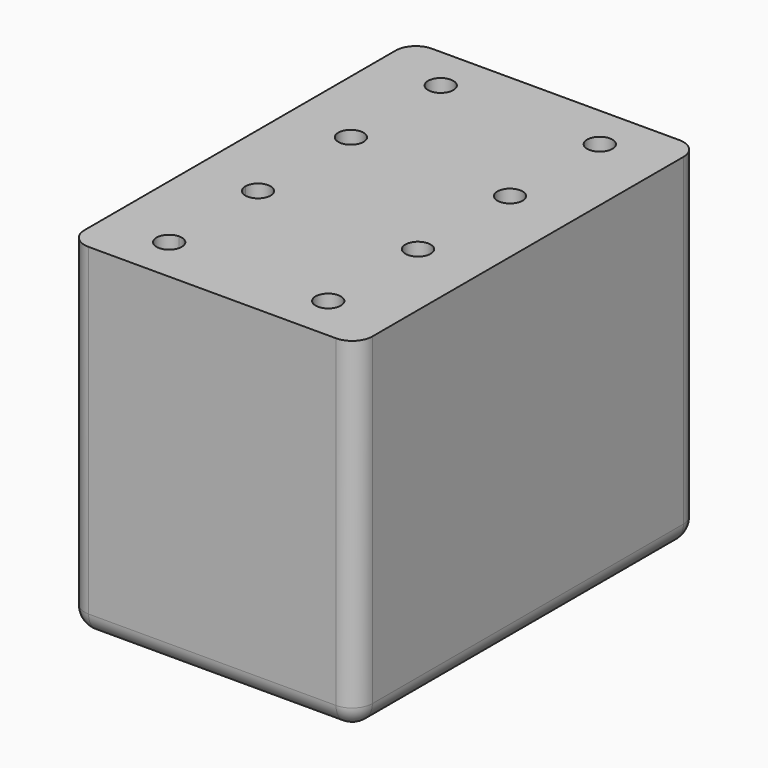
from build123d import *

# Parameters (mm, degrees)
F0_R     = 2.5
F1_DEPTH = 68
F2_R     = 4


with BuildPart() as f1:
    # F0 (on Top) → F1 (new body)
    with BuildSketch(Plane.XY):
        with BuildLine():
            Line((-44.25, -10.5), (-44.25, 0))
            Line((-44.25, 0), (-57, 0))
            Line((-57, 0), (-57, -22))
            Line((-57, -22), (0, -22))
            Line((0, -22), (0, 0))
            Line((0, 0), (-28.5, 0))
            Line((-28.5, 0), (-28.5, -13))
            Line((-28.5, -13), (-41.75, -13))
            ThreePointArc((-41.75, -13), (-46.017766953, -14.767766953), (-44.25, -10.5))
        make_face()
        with BuildLine():
            ThreePointArc((-10.25, -13), (-12.75, -15.5), (-15.25, -13))
            ThreePointArc((-15.25, -13), (-12.75, -10.5), (-10.25, -13))
        make_face(mode=Mode.SUBTRACT)
        with BuildLine():
            Line((-44.25, 6.5), (-44.25, 0))
            Line((-44.25, 0), (-28.5, 0))
            Line((-28.5, 0), (0, 0))
            Line((0, 0), (0, 63))
            Line((0, 63), (-57, 63))
            Line((-57, 63), (-57, 9))
            Line((-57, 9), (-46.75, 9))
            ThreePointArc((-46.75, 9), (-44.25, 11.5), (-41.75, 9))
            ThreePointArc((-41.75, 9), (-42.482233047, 7.232233047), (-44.25, 6.5))
        make_face()
        with Locations((-12.75, 9.2245186158)):
            Circle(F0_R, mode=Mode.SUBTRACT)
        with Locations((-44.25, 32)):
            Circle(F0_R, mode=Mode.SUBTRACT)
        with BuildLine():
            ThreePointArc((-46.75, 54.2245186158), (-44.25, 56.7245186158), (-41.75, 54.2245186158))
            ThreePointArc((-41.75, 54.2245186158), (-44.25, 51.7245186158), (-46.75, 54.2245186158))
        make_face(mode=Mode.SUBTRACT)
        with Locations((-12.75, 32)):
            Circle(F0_R, mode=Mode.SUBTRACT)
        with BuildLine():
            ThreePointArc((-15.25, 54.2245186158), (-12.75, 56.7245186158), (-10.25, 54.2245186158))
            ThreePointArc((-10.25, 54.2245186158), (-12.75, 51.7245186158), (-15.25, 54.2245186158))
        make_face(mode=Mode.SUBTRACT)
        with BuildLine():
            Line((-57, 0), (-44.25, 0))
            Line((-44.25, 0), (-44.25, 6.5))
            ThreePointArc((-44.25, 6.5), (-46.017766953, 7.232233047), (-46.75, 9))
            Line((-46.75, 9), (-57, 9))
            Line((-57, 9), (-57, 0))
        make_face()
        with BuildLine():
            Line((-28.5, 0), (-44.25, 0))
            Line((-44.25, 0), (-44.25, -10.5))
            ThreePointArc((-44.25, -10.5), (-42.482233047, -11.232233047), (-41.75, -13))
            Line((-41.75, -13), (-28.5, -13))
            Line((-28.5, -13), (-28.5, 0))
        make_face()
    extrude(amount=F1_DEPTH)

    # F2
    f2_edges = [f1.edges().sort_by_distance(p)[0] for p in [
        (-28.5, 63, 0),
        (0, 20.5, 0),
        (-57, 20.5, 0),
        (-57, 63, 34),
        (0, 63, 34),
        (-28.5, -22, 0),
        (-57, -22, 34),
        (0, -22, 34),
    ]]
    fillet(f2_edges, radius=F2_R)


solid = f1.part
